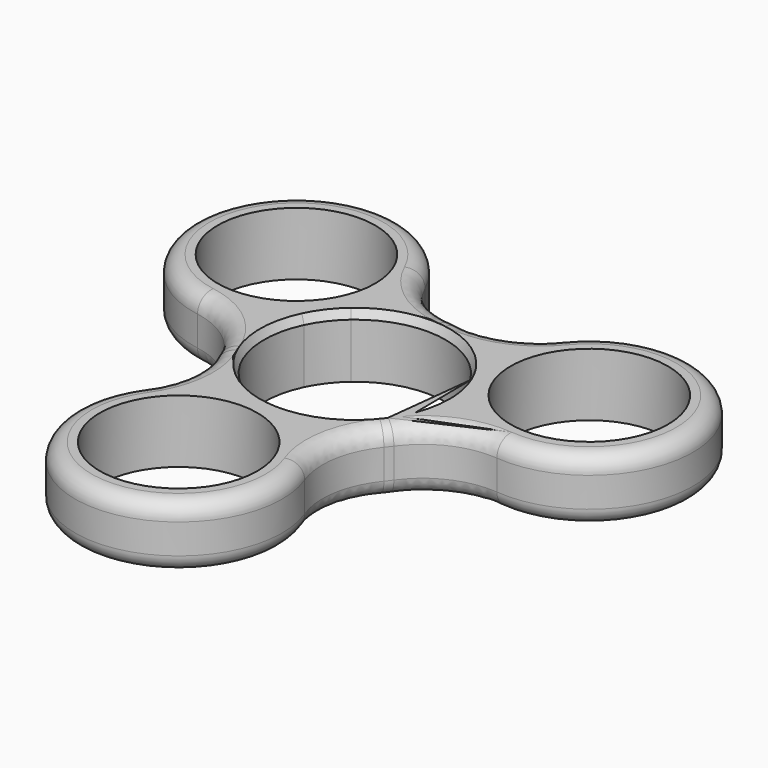
from build123d import *

# Parameters (mm, degrees)
F0_R     = 9.5
F1_DEPTH = 7.6
F2_R     = 10
F3_R     = 2
F4_SIZE2 = 0.49999
F4_SIZE  = 0.99999


# Not quite as in the source:
# - a fillet or chamfer is up to 0.001 mm smaller than in the source, because OpenCascade refuses the exact size


with BuildPart() as f1:
    # F0 (on Top) → F1 (new body)
    with BuildSketch(Plane.XY):
        with BuildLine():
            ThreePointArc((10.7678981214, 1.9886855074), (10.904379497, 0.9985027718), (10.95, 0))
            ThreePointArc((10.95, 0), (8.0413547005, -7.432302105), (0.8606640036, -10.9161237384))
            ThreePointArc((0.8606640036, -10.9161237384), (2.6908571762, -11.6770043516), (4.3777734852, -12.7176098113))
            ThreePointArc((4.3777734852, -12.7176098113), (10.668595479, -8.1904560621), (13.416858016, -0.9436212045))
            ThreePointArc((13.416858016, -0.9436212045), (11.9757710866, 0.4171928232), (10.7678981214, 1.9886855074))
        make_face()
        with BuildLine():
            ThreePointArc((9.0233084665, 6.2034187605), (10.1175075315, 4.1879041715), (10.7678981214, 1.9886855074))
            ThreePointArc((10.7678981214, 1.9886855074), (11.9757710866, 0.4171928232), (13.416858016, -0.9436212045))
            ThreePointArc((13.416858016, -0.9436212045), (13.4417119504, -0.4721015168), (13.45, 0))
            ThreePointArc((13.45, 0), (12.2392242907, 5.5770860458), (8.8248864294, 10.1500679558))
            ThreePointArc((8.8248864294, 10.1500679558), (8.7671538205, 8.1688528483), (9.0233084665, 6.2034187605))
        make_face()
        with BuildLine():
            ThreePointArc((4.3777734852, -12.7176098113), (2.6908571762, -11.6770043516), (0.8606640036, -10.9161237384))
            ThreePointArc((0.8606640036, -10.9161237384), (-1.4319223646, -10.855970631), (-3.6616968912, -10.3196160722))
            ThreePointArc((-3.6616968912, -10.3196160722), (-5.6265859601, -10.5799184025), (-7.5256289426, -11.1475292786))
            ThreePointArc((-7.5256289426, -11.1475292786), (-1.7588452789, -13.3345027386), (4.3777734852, -12.7176098113))
        make_face()
        with BuildLine():
            ThreePointArc((-7.1062012302, 8.3309305648), (1.4319223646, 10.855970631), (9.0233084665, 6.2034187605))
            ThreePointArc((9.0233084665, 6.2034187605), (8.7671538205, 8.1688528483), (8.8248864294, 10.1500679558))
            ThreePointArc((8.8248864294, 10.1500679558), (1.7588452789, 13.3345027386), (-5.8912290734, 12.0911504831))
            ThreePointArc((-5.8912290734, 12.0911504831), (-6.3491851265, 10.1627255793), (-7.1062012302, 8.3309305648))
        make_face()
        with BuildLine():
            ThreePointArc((13.45, 0), (13.4417119504, -0.4721015168), (13.416858016, -0.9436212045))
            ThreePointArc((13.416858016, -0.9436212045), (26.651311801, -2.4769444107), (33.7513856826, 8.7965110452))
            ThreePointArc((33.7513856826, 8.7965110452), (21.9291612115, 21.2781223327), (8.8248864294, 10.1500679558))
            ThreePointArc((8.8248864294, 10.1500679558), (12.2392242907, 5.5770860458), (13.45, 0))
        make_face()
        with Locations((21.2513856826, 8.7965110452)):
            Circle(F0_R, mode=Mode.SUBTRACT)
        with BuildLine():
            ThreePointArc((-7.5256289426, -11.1475292786), (-5.6265859601, -10.5799184025), (-3.6616968912, -10.3196160722))
            ThreePointArc((-3.6616968912, -10.3196160722), (-10.1175075315, -4.1879041715), (-9.8839724702, 4.7127049779))
            ThreePointArc((-9.8839724702, 4.7127049779), (-11.4580109967, 3.5081515033), (-13.2026599146, 2.5675418555))
            ThreePointArc((-13.2026599146, 2.5675418555), (-12.4274407579, -5.1440466764), (-7.5256289426, -11.1475292786))
        make_face()
        with BuildLine():
            ThreePointArc((9.4923091885, -22.8024953894), (8.1405894081, -17.1486605717), (4.3777734852, -12.7176098113))
            ThreePointArc((4.3777734852, -12.7176098113), (-1.7588452789, -13.3345027386), (-7.5256289426, -11.1475292786))
            ThreePointArc((-7.5256289426, -11.1475292786), (-10.0708265655, -33.1156963144), (9.4923091885, -22.8024953894))
        make_face()
        with Locations((-3.0076908115, -22.8024953894)):
            Circle(F0_R, mode=Mode.SUBTRACT)
        with BuildLine():
            ThreePointArc((-9.8839724702, 4.7127049779), (-8.6855851669, 6.6680664595), (-7.1062012302, 8.3309305648))
            ThreePointArc((-7.1062012302, 8.3309305648), (-6.3491851265, 10.1627255793), (-5.8912290734, 12.0911504831))
            ThreePointArc((-5.8912290734, 12.0911504831), (-10.668595479, 8.1904560621), (-13.2026599146, 2.5675418555))
            ThreePointArc((-13.2026599146, 2.5675418555), (-11.4580109967, 3.5081515033), (-9.8839724702, 4.7127049779))
        make_face()
        with BuildLine():
            ThreePointArc((-13.2026599146, 2.5675418555), (-10.668595479, 8.1904560621), (-5.8912290734, 12.0911504831))
            ThreePointArc((-5.8912290734, 12.0911504831), (-5.7806329987, 13.0457298133), (-5.7436948711, 14.0059843442))
            ThreePointArc((-5.7436948711, 14.0059843442), (-28.7141995619, 20.833760814), (-13.2026599146, 2.5675418555))
        make_face()
        with Locations((-18.2436948711, 14.0059843442)):
            Circle(F0_R, mode=Mode.SUBTRACT)
    extrude(amount=F1_DEPTH)

    # F2
    f2_edges = [f1.edges().sort_by_distance(p)[0] for p in [
        (-13.20266, 2.567542, 3.8),
        (-5.891229, 12.09115, 3.8),
        (8.824886, 10.150068, 3.8),
        (13.416858, -0.943621, 3.8),
        (4.377773, -12.71761, 3.8),
        (-7.525629, -11.147529, 3.8),
    ]]
    fillet(f2_edges, radius=F2_R)

    # F3
    f3_edges = [f1.edges().sort_by_distance(p)[0] for p in [
        (14.950396, -4.50365, 0),
        (-11.375473, -10.695598, 7.6),
    ]]
    fillet(f3_edges, radius=F3_R)

    # F4 (size 1 and 0.5 in the source; OpenCascade refuses exactly that, so slightly less here)
    f4_edges = [f1.edges().sort_by_distance(p)[0] for p in [
        (9.883972, -4.712705, 7.6),
    ]]
    f4_side = f1.faces().sort_by_distance((9.883972, -4.712705, 3.8))[0]
    chamfer(f4_edges, length=F4_SIZE, length2=F4_SIZE2, reference=f4_side)


solid = f1.part
